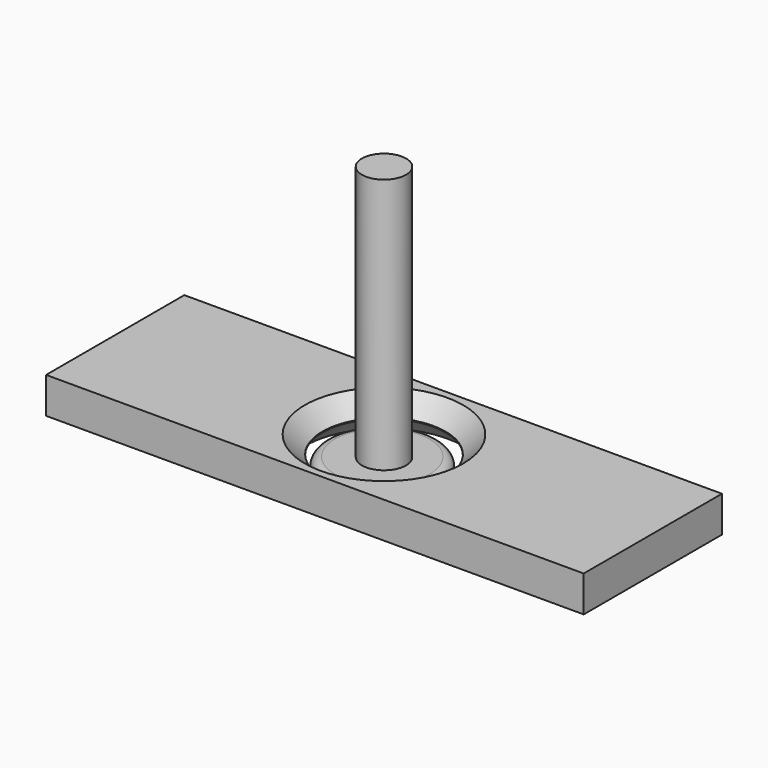
from build123d import *

# Parameters (mm, degrees)
F0_W     = 155.297530815
F0_H     = 49.9070994556
F0_R     = 17.7979211921
F1_DEPTH = 4.572
F2_W     = 155.297530815
F2_H     = 49.9070994556
F2_R     = 17.7979211921
F3_DEPTH = 5.842
F4_R     = 16.2462540438
F5_DEPTH = 4.572
F6_R     = 2.54
F8_R     = 6.3800715249
F9_DEPTH = 78.486
F10_SIZE = 5.08
F11_SIZE = 5.08


# Not quite as in the source:
# - a fillet or chamfer that OpenCascade refuses, or shapes differently, is made with other operations: its cross-section is extruded or revolved along the edge and cut away or added


with BuildPart() as f1:
    # F0 (on Top) → F1 (new body)
    with BuildSketch(Plane.XY):
        Rectangle(F0_W, F0_H)
        Circle(F0_R, mode=Mode.SUBTRACT)
    extrude(amount=F1_DEPTH)

    # F2 (on face) → F3 (join)
    with BuildSketch(Plane.XY.offset(4.572)):
        Rectangle(F2_W, F2_H)
        Circle(F2_R, mode=Mode.SUBTRACT)
    extrude(amount=F3_DEPTH)

    # F10
    f10_edges = [f1.edges().sort_by_distance(p)[0] for p in [
        (-17.797921, 0, 0),
    ]]
    chamfer(f10_edges, length=F10_SIZE)

    # F11
    f11_edges = [f1.edges().sort_by_distance(p)[0] for p in [
        (-17.797921, 0, 10.414),
    ]]
    chamfer(f11_edges, length=F11_SIZE)


with BuildPart() as f5:
    # F4 (on Top) → F5 (new body)
    with BuildSketch(Plane.XY):
        with Locations((-0.5184755428, 0)):
            Circle(F4_R)
    extrude(amount=F5_DEPTH)

    # F6
    f6_edges = [f5.edges().sort_by_distance(p)[0] for p in [
        (-16.76473, 0, 4.572),
    ]]
    fillet(f6_edges, radius=F6_R)

    # F7: fillet of radius 2.54 on 1 edges, made by hand

    # F7_s1 → F7_t2 (revolve, cut)
    with BuildSketch(Plane.XZ):
        with BuildLine():
            ThreePointArc((15.7277785011, 2.032), (14.8455339738, 0.5725244601), (13.2390969224, 0))
            Line((13.2390969224, 0), (15.7277785011, 0))
            Line((15.7277785011, 0), (15.7277785011, 2.032))
        make_face()
    revolve(axis=Axis((-0.5184755428, 0, 0), (0, 0, 1)), mode=Mode.SUBTRACT)


with BuildPart() as f9:
    # F8 (on Top) → F9 (new body)
    with BuildSketch(Plane.XY):
        Circle(F8_R)
    extrude(amount=F9_DEPTH)


solid = Compound([f1.part, f5.part, f9.part])
